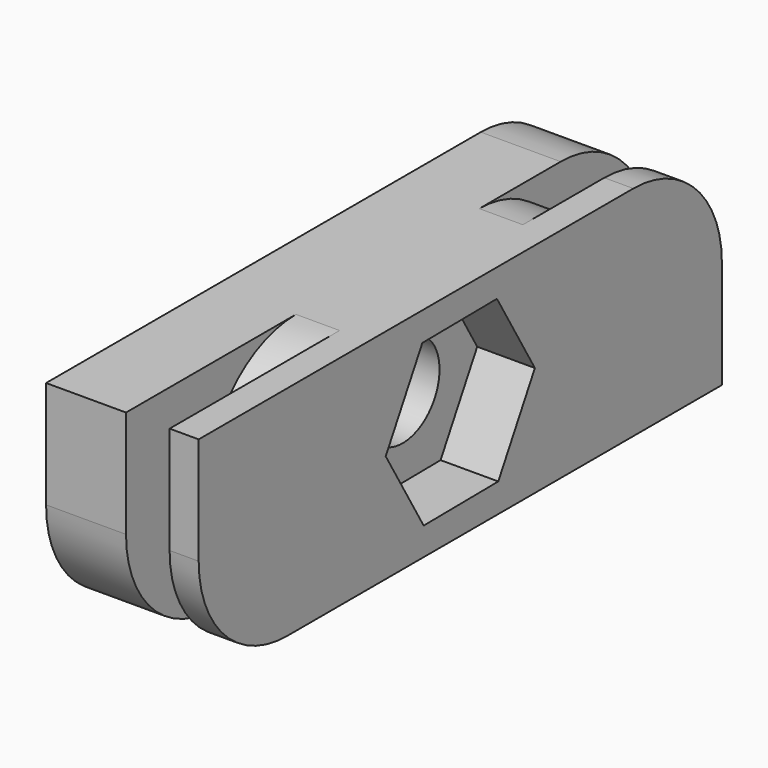
from build123d import *

# Parameters (mm, degrees)
F1_DEPTH    = 15
F2_R        = 3.175
F3_DEPTH    = 25.4
F4_R        = 3.175
F5_DEPTH    = 3.96875
F6_T1_DEPTH = 3
F7_R        = 7.62


# Not quite as in the source:
# - a fillet or chamfer that OpenCascade refuses, or shapes differently, is made with other operations: its cross-section is extruded or revolved along the edge and cut away or added


with BuildPart() as f1:
    # F0 (on Top) → F1 (new body)
    with BuildSketch(Plane.XY):
        Polygon((-23.4638472274, 38), (-23.4638472274, -7), (-17.9638472274, -7), (-17.9638472274, 0), (-14.9638472274, 0), (-14.9638472274, -7), (-12.9638472274, -7), (-12.9638472274, 38), (-14.9638472274, 38), (-14.9638472274, 31), (-17.9638472274, 31), (-17.9638472274, 38), align=None)
    extrude(amount=F1_DEPTH)

    # F2 (on face) → F3 (cut)
    with BuildSketch(Plane(origin=(-23.4638472274, 0, 0), x_dir=(0, -1, 0), z_dir=(-1, 0, 0))):
        with Locations((-15.5, 7.5)):
            Circle(F2_R)
    extrude(amount=-F3_DEPTH, mode=Mode.SUBTRACT)

    # F4 (on face) → F5 (cut)
    with BuildSketch(Plane.YZ.offset(-12.9638472274)):
        Polygon((21.9154598913, 7.5665316996), (18.6501118036, 13.0892170926), (12.2346519124, 13.022685393), (9.0845401087, 7.4334683004), (12.3498881964, 1.9107829074), (18.7653480876, 1.977314607), align=None)
        with Locations((15.5, 7.5)):
            Circle(F4_R, mode=Mode.SUBTRACT)
    extrude(amount=-F5_DEPTH, mode=Mode.SUBTRACT)

    # F6: fillet of radius 7.62 on 4 edges, made by hand

    # F6_s2 → F6_t1 (cut)
    with BuildSketch(Plane.YZ.offset(-17.9638472274)):
        with BuildLine():
            ThreePointArc((7.62, 15), (2.2318463274, 12.7681536726), (0, 7.38))
            Line((0, 7.38), (-0.1524, 7.38))
            Line((-0.1524, 7.38), (-0.1524, 15.1524))
            Line((-0.1524, 15.1524), (7.62, 15.1524))
            Line((7.62, 15.1524), (7.62, 15))
        make_face()
        with BuildLine():
            ThreePointArc((23.38, 15), (28.7681536726, 12.7681536726), (31, 7.38))
            Line((31, 7.38), (31.1524, 7.38))
            Line((31.1524, 7.38), (31.1524, 15.1524))
            Line((31.1524, 15.1524), (23.38, 15.1524))
            Line((23.38, 15.1524), (23.38, 15))
        make_face()
        with BuildLine():
            ThreePointArc((0, 7.62), (2.2318463274, 2.2318463274), (7.62, 0))
            Line((7.62, 0), (7.62, -0.1524))
            Line((7.62, -0.1524), (-0.1524, -0.1524))
            Line((-0.1524, -0.1524), (-0.1524, 7.62))
            Line((-0.1524, 7.62), (0, 7.62))
        make_face()
        with BuildLine():
            ThreePointArc((31, 7.62), (28.7681536726, 2.2318463274), (23.38, 0))
            Line((23.38, 0), (23.38, -0.1524))
            Line((23.38, -0.1524), (31.1524, -0.1524))
            Line((31.1524, -0.1524), (31.1524, 7.62))
            Line((31.1524, 7.62), (31, 7.62))
        make_face()
    extrude(amount=F6_T1_DEPTH, mode=Mode.SUBTRACT)

    # F7
    f7_edges = [f1.edges().sort_by_distance(p)[0] for p in [
        (-13.963847, 38, 15),
        (-13.963847, -7, 0),
        (-20.713847, -7, 0),
        (-20.713847, 38, 15),
    ]]
    fillet(f7_edges, radius=F7_R)


solid = f1.part
